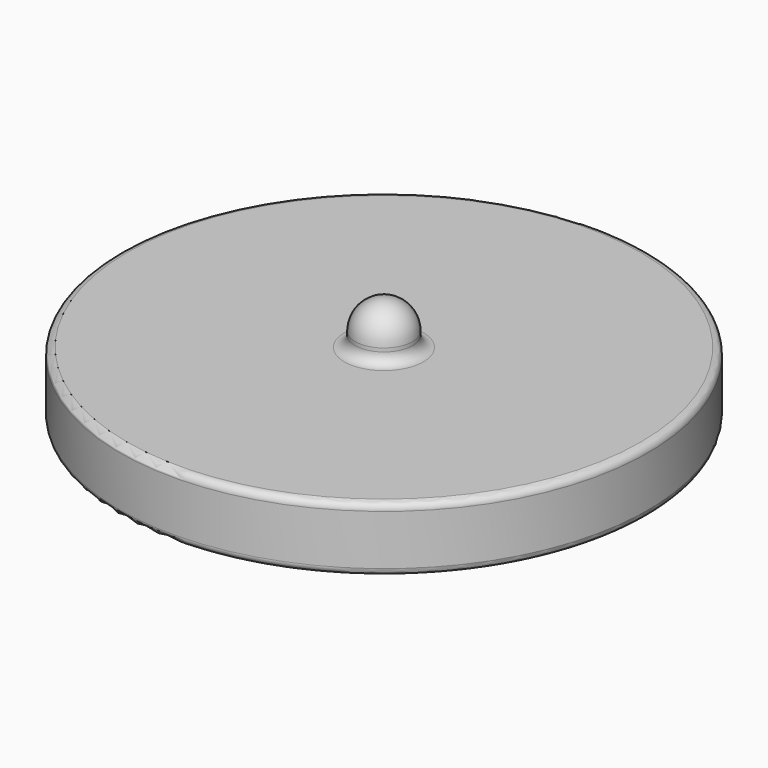
from build123d import *

# Parameters (mm, degrees)
F0_W = 0.8
F0_H = 0.4
F2_R = 0.2
F3_R = 0.3


# Not quite as in the source:
# - a feature names something its author has since deleted; it is built from what else it names


with BuildPart() as f1:
    # F0 (on Front) → F1 (revolve)
    with BuildSketch(Plane.XZ):
        Polygon((-6.35, 0), (0, 0), (0, 1), (-0.8, 1), (-7.35, 1), (-7.35, -0.8), (-6.35, -0.8), align=None)
        with Locations((-0.4, 1.2)):
            Rectangle(F0_W, F0_H)
        with BuildLine():
            Line((-0.8, 1.4), (0, 1.4))
            Line((0, 1.4), (0, 2.2))
            ThreePointArc((0, 2.2), (-0.5656854249, 1.9656854249), (-0.8, 1.4))
        make_face()
    revolve(axis=Axis((0, 0, 0.5), (0, 0, 1)))

    # F2
    f2_edges = [f1.edges().sort_by_distance(p)[0] for p in [
        (7.35, 0, 1),
        (7.35, 0, -0.8),
        (6.35, 0, -0.8),
    ]]
    fillet(f2_edges, radius=F2_R)

    # F3
    f3_edges = [f1.edges().sort_by_distance(p)[0] for p in [
        (0.8, 0, 1),
    ]]
    fillet(f3_edges, radius=F3_R)


solid = f1.part
